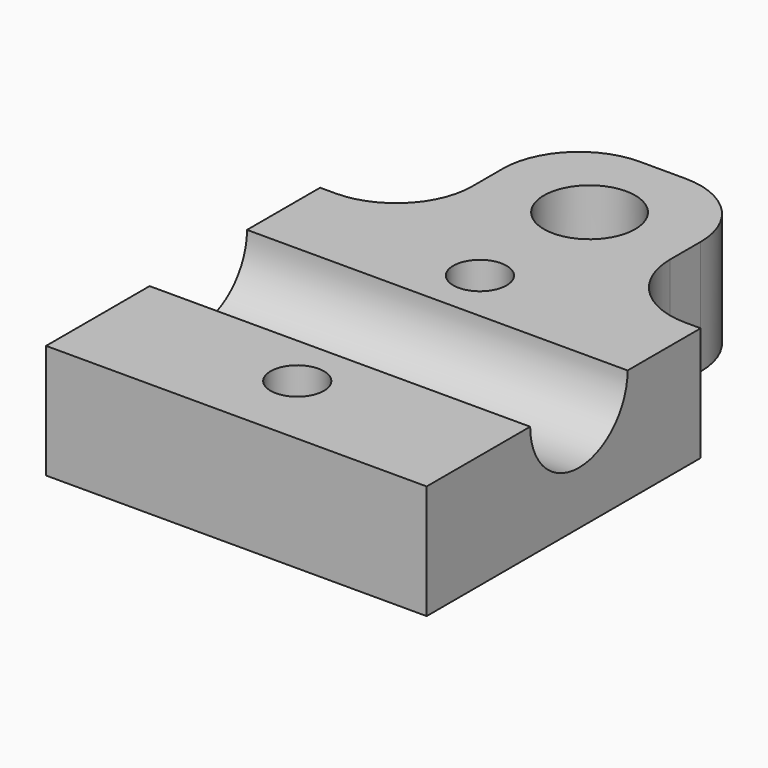
from build123d import *

# Parameters (mm, degrees)
F0_W     = 50
F0_H     = 70
F1_DEPTH = 15
F2_R     = 6
F3_DEPTH = 25
F4_R     = 8
F5_DEPTH = 50.001
F6_R     = 3.5
F7_DEPTH = 15.001
F8_W     = 12
F8_H     = 25
F9_DEPTH = 15
F10_R    = 10


# Not quite as in the source:
# - a feature names something its author has since deleted; it is built from what else it names


with BuildPart() as f1:
    # F0 (on Top) → F1 (new body)
    with BuildSketch(Plane.XY):
        with Locations((6.2123397365, -48.3642113331)):
            Rectangle(F0_W, F0_H)
    extrude(amount=F1_DEPTH)

    # F2 (on face) → F3 (cut)
    with BuildSketch(Plane.XY.offset(15)):
        with Locations((6.2123397365, -25.3642113331)):
            Circle(F2_R)
    extrude(amount=-F3_DEPTH, mode=Mode.SUBTRACT)

    # F4 (on face) → F5 (cut, through all)
    with BuildSketch(Plane.YZ.offset(31.2123397365)):
        with Locations((-58.3642113331, 15)):
            Circle(F4_R)
    extrude(amount=-F5_DEPTH, mode=Mode.SUBTRACT)

    # F6 (on face) → F7 (cut, through all)
    with BuildSketch(Plane(origin=(0, 0, 0), x_dir=(1, 0, 0), z_dir=(0, 0, -1))):
        with Locations((6.2123397365, 43.3642113331)):
            Circle(F6_R)
        with Locations((6.2123397365, 73.3642113331)):
            Circle(F6_R)
    extrude(amount=-F7_DEPTH, mode=Mode.SUBTRACT)

    # F8 (on face) → F9 (cut, through all)
    with BuildSketch(Plane.XY.offset(15)):
        with Locations((25.2123397365, -25.8642113331)):
            Rectangle(F8_W, F8_H)
        with Locations((-12.7876602635, -25.8642113331)):
            Rectangle(F8_W, F8_H)
    extrude(amount=-F9_DEPTH, mode=Mode.SUBTRACT)

    # F10
    f10_edges = [f1.edges().sort_by_distance(p)[0] for p in [
        (19.21234, -13.364211, 7.5),
        (-6.78766, -13.364211, 7.5),
        (-6.78766, -38.364211, 7.5),
        (19.21234, -38.364211, 7.5),
    ]]
    fillet(f10_edges, radius=F10_R)


solid = f1.part
